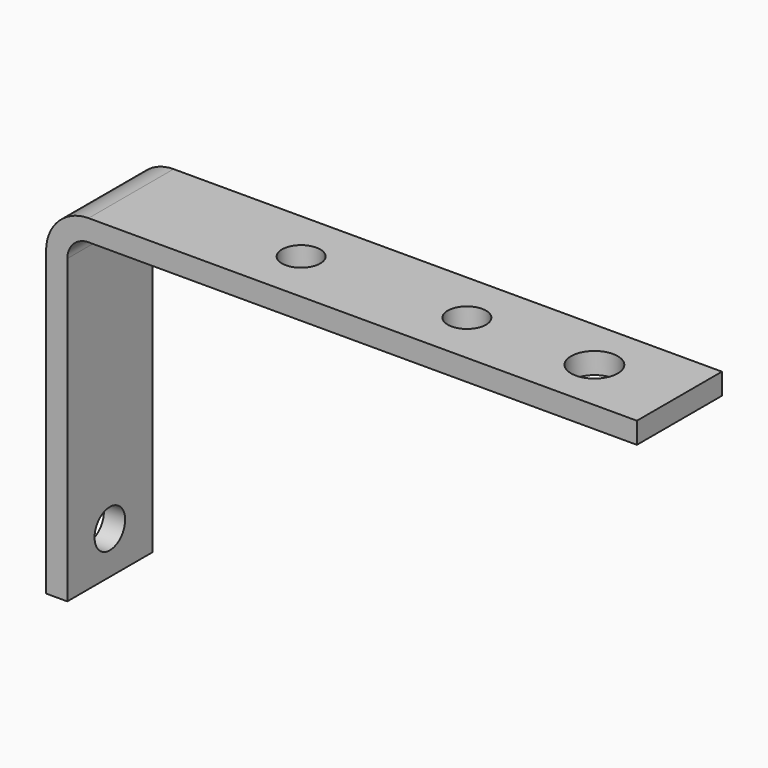
from build123d import *

# Parameters (mm, degrees)
F1_DEPTH = 25
F2_R     = 5.5
F2_R_2   = 4.5
F3_DEPTH = 5
F4_DEPTH = 5
F5_R     = 4.5
F6_DEPTH = 5


# Not quite as in the source:
# - ends of sketch curves that miss each other by under 0.0002 mm in the source are joined


with BuildPart() as f1:
    # F0 (on Front) → F1 (new body)
    with BuildSketch(Plane.XZ):
        with BuildLine():
            Line((134, 0), (134, 5))
            Line((134, 5), (5, 5))
            ThreePointArc((5, 5), (2.4118095455, 4.6592580848), (0, 3.6602538402))
            Line((0, 3.6602538402), (0, 0))
            Line((0, 0), (5, 0))
            Line((5, 0), (134, 0))
        make_face()
        with BuildLine():
            Line((0, 0), (0, 3.6602538402))
            ThreePointArc((0, 3.6602538402), (-3.6602539143, -1.284e-07), (-4.9999998289, -5))
            Line((-4.9999998289, -5), (-5, -76))
            Line((-5, -76), (0, -76))
            Line((0, -76), (0, -5))
            Line((0, -5), (0, 0))
        make_face()
        with BuildLine():
            ThreePointArc((0, -5), (1.4644660941, -1.4644660941), (5, 0))
            Line((5, 0), (0, 0))
            Line((0, 0), (0, -5))
        make_face()
    extrude(amount=-F1_DEPTH)

    # F2 (on face) → F3 (cut)
    with BuildSketch(Plane.XY.offset(5)):
        with Locations((114, 12.5)):
            Circle(F2_R)
        with Locations((84, 12.5)):
            Circle(F2_R_2)
        with Locations((45, 12.5)):
            Circle(F2_R_2)
    extrude(amount=-F3_DEPTH, mode=Mode.SUBTRACT)

    # F2 (on face) → F4 (cut)
    with BuildSketch(Plane.XY.offset(5)):
        with Locations((114, 12.5)):
            Circle(F2_R)
        with Locations((84, 12.5)):
            Circle(F2_R_2)
        with Locations((45, 12.5)):
            Circle(F2_R_2)
    extrude(amount=-F4_DEPTH, mode=Mode.SUBTRACT)

    # F5 (on face) → F6 (cut)
    with BuildSketch(Plane(origin=(-5, 0, 0), x_dir=(0, -1, 0), z_dir=(-1, 0, 0))):
        with Locations((-12.5, -66)):
            Circle(F5_R)
    extrude(amount=-F6_DEPTH, mode=Mode.SUBTRACT)


solid = f1.part
